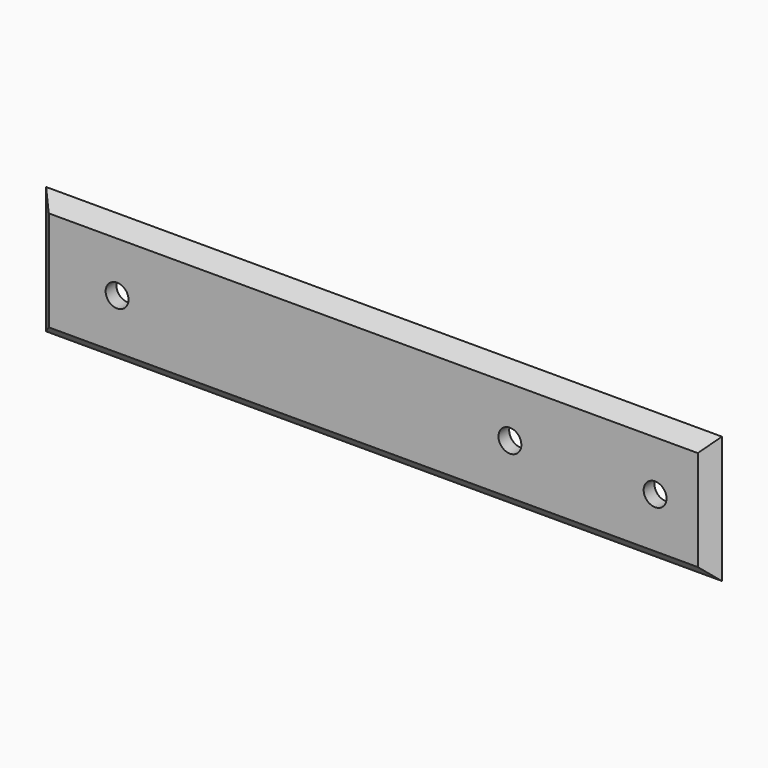
from build123d import *

# Parameters (mm, degrees)
F1_DEPTH    = 3.9878
F2_T1_DEPTH = 229.3282991577
F2_T3_DEPTH = 66.1332991577


# Not quite as in the source:
# - a fillet or chamfer that OpenCascade refuses, or shapes differently, is made with other operations: its cross-section is extruded or revolved along the edge and cut away or added


with BuildPart() as f1:
    # F0 (on Front) → F1 (new body)
    with BuildSketch(Plane.XZ):
        with BuildLine():
            Line((0, -20.0025), (101.6, -20.0025))
            Line((101.6, -20.0025), (101.6, 0))
            Line((101.6, 0), (87.21852, 0))
            ThreePointArc((87.21852, 0), (83.82, -3.39852), (80.42148, 0))
            Line((80.42148, 0), (44.0436, 0))
            ThreePointArc((44.0436, 0), (40.64, -3.4036), (37.2364, 0))
            Line((37.2364, 0), (0, 0))
            Line((0, 0), (0, -20.0025))
        make_face()
        Polygon((-101.6, -20.0025), (0, -20.0025), (0, 0), (0, 20.0025), (-101.6, 20.0025), (-101.6, 0), align=None)
        with BuildLine():
            ThreePointArc((-72.80148, 0), (-76.2, -3.39852), (-79.59852, 0))
            ThreePointArc((-79.59852, 0), (-76.2, 3.39852), (-72.80148, 0))
        make_face(mode=Mode.SUBTRACT)
        with BuildLine():
            Line((87.21852, 0), (101.6, 0))
            Line((101.6, 0), (101.6, 20.0025))
            Line((101.6, 20.0025), (0, 20.0025))
            Line((0, 20.0025), (0, 0))
            Line((0, 0), (37.2364, 0))
            ThreePointArc((37.2364, 0), (40.64, 3.4036), (44.0436, 0))
            Line((44.0436, 0), (80.42148, 0))
            ThreePointArc((80.42148, 0), (83.82, 3.39852), (87.21852, 0))
        make_face()
    extrude(amount=F1_DEPTH)

    # F2: chamfer of 5.08 on 4 edges, made by hand

    # F2_s2 → F2_t1 (cut)
    with BuildSketch(Plane.YZ.offset(-114.6641495789)):
        Polygon((1.0922, 20.0025), (-3.9878, 14.9225), (-3.9878, 20.0025), align=None)
        Polygon((1.0922, -20.0025), (-3.9878, -14.9225), (-3.9878, -20.0025), align=None)
    extrude(amount=F2_T1_DEPTH, mode=Mode.SUBTRACT)

    # F2_s4 → F2_t3 (cut)
    with BuildSketch(Plane.XY.offset(-33.0666495789)):
        Polygon((-101.6, 1.0922), (-96.52, -3.9878), (-101.6, -3.9878), align=None)
        Polygon((101.6, 1.0922), (96.52, -3.9878), (101.6, -3.9878), align=None)
    extrude(amount=F2_T3_DEPTH, mode=Mode.SUBTRACT)


solid = f1.part
